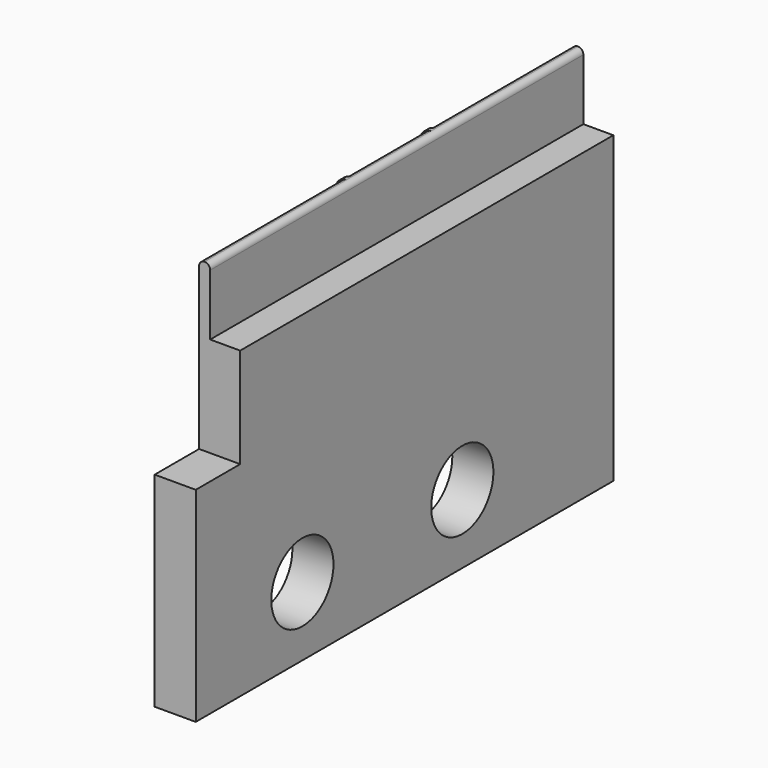
from build123d import *

# Parameters (mm, degrees)
F1_DEPTH = 1.85
F2_W     = 0.5
F2_H     = 21
F3_DEPTH = 3
F4_R     = 1.75
F5_DEPTH = 1.851
F6_W     = 0.25
F6_H     = 3.7
F7_DEPTH = 0.25
F8_R     = 0.24999
F9_R     = 0.4999
F10_R    = 0.24999


# Not quite as in the source:
# - a fillet or chamfer is up to 0.001 mm smaller than in the source, because OpenCascade refuses the exact size


with BuildPart() as f1:
    # F0 (on Right) → F1 (new body)
    with BuildSketch(Plane.YZ):
        Polygon((0, 9.2), (0, 0), (23.5, 0), (23.5, 13.7), (2.5, 13.7), (2.5, 9.2), align=None)
    extrude(amount=F1_DEPTH)

    # F2 (on face) → F3 (join)
    with BuildSketch(Plane.XY.offset(13.7)):
        with Locations((0.25, 13)):
            Rectangle(F2_W, F2_H)
    extrude(amount=F3_DEPTH)

    # F4 (on face) → F5 (cut, through all)
    with BuildSketch(Plane.YZ.offset(1.85)):
        with Locations((6, 3.1)):
            Circle(F4_R)
        with Locations((15, 3.1)):
            Circle(F4_R)
    extrude(amount=-F5_DEPTH, mode=Mode.SUBTRACT)

    # F6 (on face) → F7 (join)
    with BuildSketch(Plane(origin=(0, 0, 0), x_dir=(0, -1, 0), z_dir=(-1, 0, 0))):
        with Locations((-15.375, 14.85)):
            Rectangle(F6_W, F6_H)
        with Locations((-10.625, 14.85)):
            Rectangle(F6_W, F6_H)
    extrude(amount=F7_DEPTH)

    # F8 (radius 0.25 in the source; OpenCascade refuses exactly that, so slightly less here)
    f8_edges = [f1.edges().sort_by_distance(p)[0] for p in [
        (0, 6.5, 16.7),
        (0, 13, 16.7),
        (0, 19.5, 16.7),
        (0.5, 13, 16.7),
    ]]
    fillet(f8_edges, radius=F8_R)

    # F9 (radius 0.5 in the source; OpenCascade refuses exactly that, so slightly less here)
    f9_edges = [f1.edges().sort_by_distance(p)[0] for p in [
        (-0.25, 15.375, 16.7),
        (-0.25, 10.625, 16.7),
    ]]
    fillet(f9_edges, radius=F9_R)

    # F10 (radius 0.25 in the source; OpenCascade refuses exactly that, so slightly less here)
    f10_edges = [f1.edges().sort_by_distance(p)[0] for p in [
        (-0.25, 10.625, 13),
        (-0.25, 15.375, 13),
    ]]
    fillet(f10_edges, radius=F10_R)


solid = f1.part
